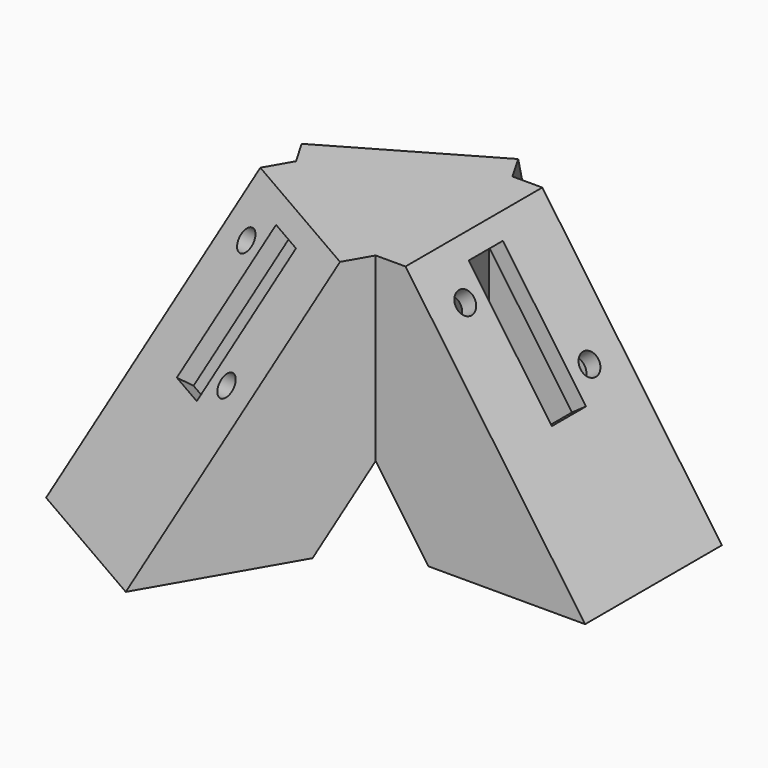
from build123d import *

# Parameters (mm, degrees)
F1_DEPTH        = 12.7
F3_COUNT        = 3
F4_T            = 2.54
F4_T3_DEPTH     = 31.9573897847
F5_W            = 6.35
F5_H            = 21.5367313986
F5_R            = 1.651
F6_DEPTH        = 2.54
F6_COPIES_COUNT = 3


# Not quite as in the source:
# - a pattern or mirror of a feature is missing from the dataset's text; its kind, count and spacing are read off the source's solid
# - a shell that OpenCascade refuses in one call is made with other operations: the cavity is built on its own and cut out


with BuildPart() as f1:
    # F0 (on Front) → F1 (new body, symmetric)
    with BuildSketch(Plane.XZ):
        Polygon((11.7683534, 0), (0, 0), (0, -16.4057110057), (15.1905046899, -38.1), (38.4462606058, -38.1), align=None)
    extrude(amount=F1_DEPTH, both=True)

    # F3: F1 ×3 about axis
    f3_axis = Axis((0, 0, -8.2028555029), (0, 0, -1))


with BuildPart() as f1_1:
    add(f1.part)
    for i in range(1, F3_COUNT):
        add(f1.part.rotate(f3_axis, i * 360 / F3_COUNT))

    # F4: shell of thickness 2.54, made by hand


with BuildPart() as f4_core1:
    # F4_t2: copy of F1
    add(f1_1.part)

    # the walls: a layer under each face that stays
    f4_faces = [f4_core1.faces().sort_by_distance(p)[0] for p in [
        (-2.557172964, 0, 0),
        (22.8893045122, -12.7, -19.05),
        (-0.4461296281, -26.1727191826, -19.05),
        (-12.5536535014, -21.7435656851, -19.05),
        (-22.4431748842, -13.4727191826, -19.05),
        (22.8893045122, 12.7, -19.05),
        (25.1073070029, 0, -19.05),
        (-22.4431748842, 13.4727191826, -19.05),
        (-0.4461296281, 26.1727191826, -19.05),
        (-12.5536535014, 21.7435656851, -19.05),
    ]]
    thicken(f4_faces, amount=-F4_T, mode=Mode.SUBTRACT)

    # F4_s4 → F4_t3 (cut)
    with BuildSketch(Plane.XY.offset(-29.4173897847)):
        Polygon((7.354345464, -12.7381), (7.3323484187, -10.16), (5.865878735, -10.16), (5.1326438931, -11.43), align=None)
        Polygon((-14.7086909279, 0), (-12.4649923118, -1.27), (-11.7317574699, 0), (-12.4649923118, 1.27), align=None)
        Polygon((7.354345464, 12.7381), (7.3323484187, 10.16), (5.865878735, 10.16), (5.1326438931, 11.43), align=None)
    extrude(amount=F4_T3_DEPTH, mode=Mode.SUBTRACT)


with BuildPart() as f1_2:
    add(f1_1.part)

    # what is left inside the walls is the cavity
    f4_cavity = [f4_core1.part.solids().sort_by_distance(p)[0] for p in [
        (22.874997, 3.386667, -20.334569),
    ]]
    add(f4_cavity, mode=Mode.SUBTRACT)

    # F5 (on face) → F6 (cut)
    with BuildSketch(Plane(origin=(7.8966836583, 0, 5.5293174244), x_dir=(0, 1, 0), z_dir=(0.8191520443, 0, 0.5735764364))):
        with Locations((0, -20.5930502049)):
            Rectangle(F5_W, F5_H)
        with Locations((6.7175144213, -27.3105646262)):
            Circle(F5_R)
        with Locations((-6.7175144213, -13.8755357836)):
            Circle(F5_R)
    f6 = extrude(amount=-F6_DEPTH, mode=Mode.SUBTRACT)

    # F6_copies: F6 ×3 about axis
    f6_copies_axis = Axis((0, 0, 0), (0, 0, 1))
    for i in range(1, F6_COPIES_COUNT):
        add(f6.rotate(f6_copies_axis, i * 360 / F6_COPIES_COUNT), mode=Mode.SUBTRACT)


solid = f1_2.part
